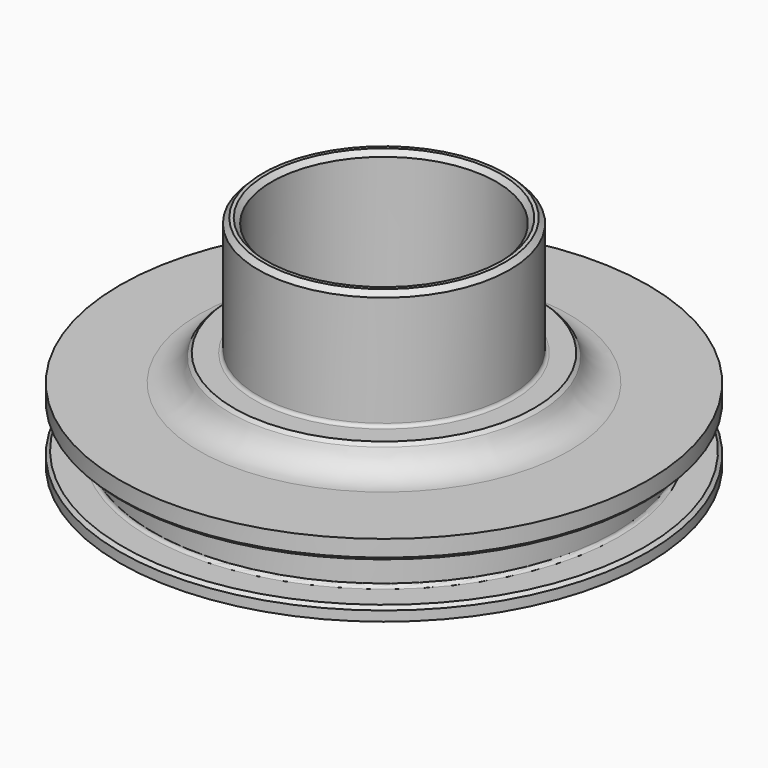
from build123d import *

# Parameters (mm, degrees)
F2_SIZE = 2
F3_SIZE = 0.75
F4_SIZE = 0.5
F5_R    = 0.5


# Not quite as in the source:
# - a fillet or chamfer that OpenCascade refuses, or shapes differently, is made with other operations: its cross-section is extruded or revolved along the edge and cut away or added


with BuildPart() as f1:
    # F0 (on Front) → F1 (revolve)
    with BuildSketch(Plane.XZ):
        Polygon((17.025, 33.05), (17.025, 0), (40, 0), (40, 2), (35, 2), (35, 8.05), (40, 8.05), (40, 11.05), (23.25, 11.05), (23.25, 15.05), (19.059525, 15.05), (19.059525, 33.05), align=None)
    revolve(axis=Axis((0, 0, 13.9434672892), (0, 0, 1)))

    # F2
    f2_edges = [f1.edges().sort_by_distance(p)[0] for p in [
        (-17.025, 0, 0),
    ]]
    chamfer(f2_edges, length=F2_SIZE)

    # F3
    f3_edges = [f1.edges().sort_by_distance(p)[0] for p in [
        (-17.025, 0, 33.05),
        (-19.059525, 0, 33.05),
    ]]
    chamfer(f3_edges, length=F3_SIZE)

    # F4
    f4_edges = [f1.edges().sort_by_distance(p)[0] for p in [
        (-23.25, 0, 15.05),
        (-40, 0, 8.05),
        (-40, 0, 2),
    ]]
    chamfer(f4_edges, length=F4_SIZE)

    # F5
    f5_edges = [f1.edges().sort_by_distance(p)[0] for p in [
        (-35, 0, 8.05),
        (-35, 0, 2),
        (-19.059525, 0, 15.05),
    ]]
    fillet(f5_edges, radius=F5_R)

    # F6: fillet of radius 5 on 1 edges, made by hand

    # F6_s1 → F6_t2 (revolve)
    with BuildSketch(Plane.XZ):
        with BuildLine():
            ThreePointArc((28.0196960071, 11.05), (25.0616561155, 12.0188711259), (23.25, 14.55))
            Line((23.25, 14.55), (23.1546060799, 14.52))
            ThreePointArc((23.1546060799, 14.52), (23.15, 12.8), (23.15, 11.05))
            Line((23.15, 11.05), (23.25, 10.95))
            Line((23.25, 10.95), (28.0196960071, 10.95))
            Line((28.0196960071, 10.95), (28.0196960071, 11.05))
        make_face()
    revolve(axis=Axis((0, 0, 11.05), (0, 0, 1)))


solid = f1.part
